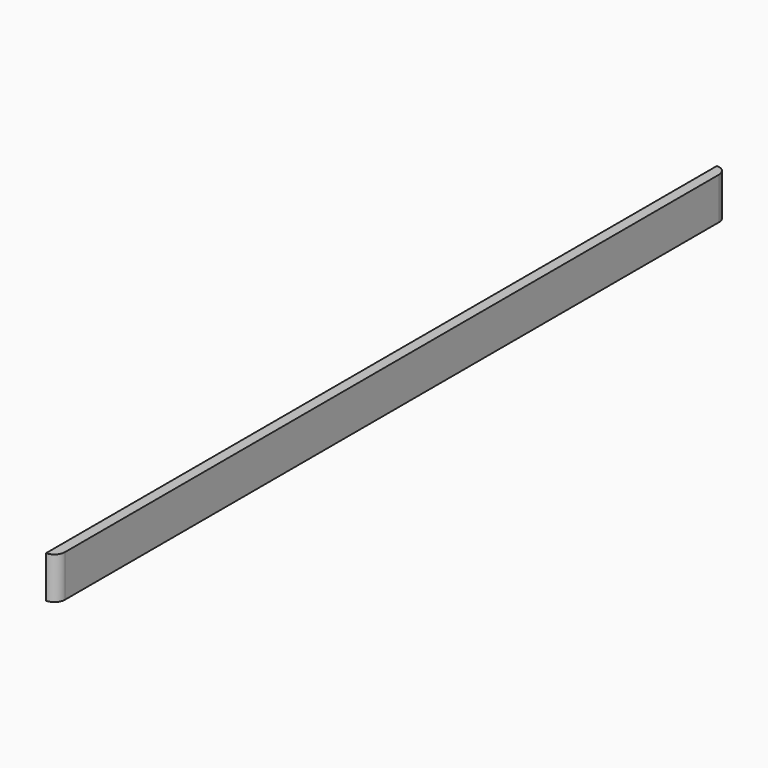
from build123d import *

# Parameters (mm, degrees)
F0_W     = 12.7
F0_H     = 50.8
F1_DEPTH = 508
F2_R     = 12.69999


# Not quite as in the source:
# - a fillet or chamfer is up to 0.001 mm smaller than in the source, because OpenCascade refuses the exact size


with BuildPart() as f1:
    # F0 (on Front) → F1 (new body, symmetric)
    with BuildSketch(Plane.XZ):
        with Locations((6.35, -25.4)):
            Rectangle(F0_W, F0_H)
    extrude(amount=F1_DEPTH, both=True)

    # F2 (radius 12.7 in the source; OpenCascade refuses exactly that, so slightly less here)
    f2_edges = [f1.edges().sort_by_distance(p)[0] for p in [
        (12.7, -508, -25.4),
        (12.7, 508, -25.4),
    ]]
    fillet(f2_edges, radius=F2_R)


solid = f1.part
